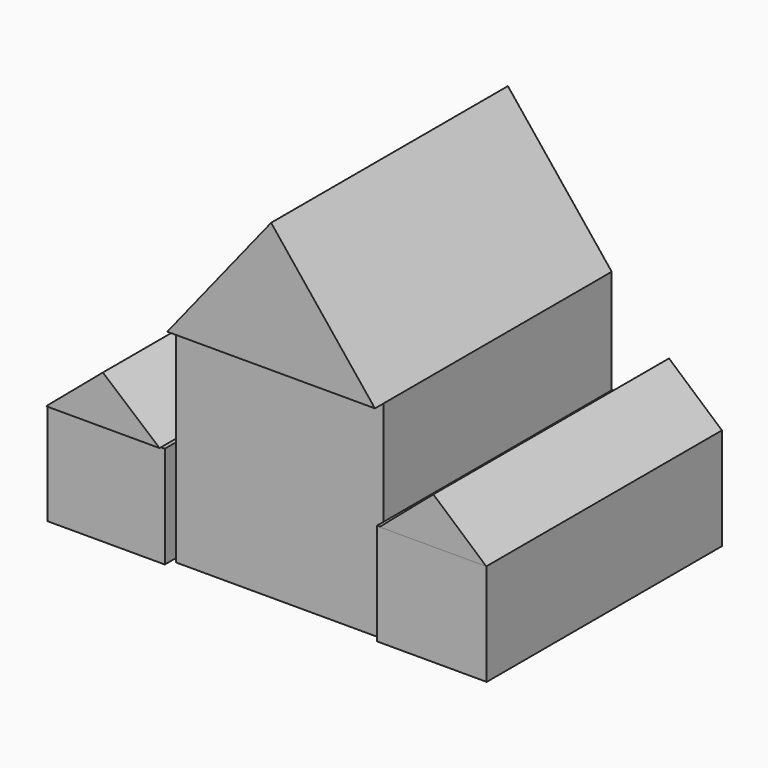
from build123d import *

# Parameters (mm, degrees)
F0_W      = 63.5
F0_H      = 63.5
F1_DEPTH  = 90.51564
F3_W      = 10.2954022586
F3_H      = 21.1791172624
F4_DEPTH  = 1.27
F6_W      = 6.7655518651
F6_H      = 6.3243201002
F7_DEPTH  = 5.08
F8_W      = 35.8868353069
F8_H      = 31.1803687364
F9_DEPTH  = 90.5202
F12_W     = 33.533602953
F12_H     = 31.1803687364
F13_DEPTH = 89.9029
F17_DEPTH = 90.07895
F19_DEPTH = 91.04824
F2_W      = 63.5
F2_H      = 63.5
F22_DEPTH = 3.36136


# Not quite as in the source:
# - the program builds the solid bodies; features that only make, move or delete a surface that nothing else refers to are left out


with BuildPart() as f1:
    # F0 (on Front) → F1 (new body)
    with BuildSketch(Plane.XZ):
        Polygon((-31.75, 31.75), (31.75, 31.75), (0, 71.4057372898), align=None)
        Rectangle(F0_W, F0_H)
    extrude(amount=F1_DEPTH)

    # F3 (on face) → F4 (cut)
    with BuildSketch(Plane.XZ.offset(90.51564)):
        with Locations((0, -20.0025010854)):
            Rectangle(F3_W, F3_H)
    extrude(amount=-F4_DEPTH, mode=Mode.SUBTRACT)

    # F6 (on face) → F7 (cut)
    with BuildSketch(Plane(origin=(-31.75, 0, 0), x_dir=(0, -1, 0), z_dir=(-1, 0, 0))):
        with Locations((15.6882982701, 15.3695684858)):
            Rectangle(F6_W, F6_H)
        with Locations((22.4538501352, 15.3695684858)):
            Rectangle(F6_W, F6_H)
        with Locations((22.4538501352, 9.0452483855)):
            Rectangle(F6_W, F6_H)
        with Locations((15.6882982701, 9.0452483855)):
            Rectangle(F6_W, F6_H)
    extrude(amount=-F7_DEPTH, mode=Mode.SUBTRACT)

    # F2 (on face) → F22 (cut)
    with BuildSketch(Plane.XZ.offset(90.51564)):
        Rectangle(F2_W, F2_H)
    extrude(amount=-F22_DEPTH, mode=Mode.SUBTRACT)


with BuildPart() as f9:
    # F8 (on Front) → F9 (new body)
    with BuildSketch(Plane.XZ):
        with Locations((-50.4474807531, -15.5901843682)):
            Rectangle(F8_W, F8_H)
    extrude(amount=F9_DEPTH)

    # F18 (on Front) → F19 (join)
    with BuildSketch(Plane.XZ):
        Polygon((-51.0357916355, 14.7077208385), (-68.3908984065, 0), (-33.6806811392, 0), align=None)
    extrude(amount=F19_DEPTH)


with BuildPart() as f13:
    # F12 (on Front) → F13 (new body)
    with BuildSketch(Plane.XZ):
        with Locations((48.6825555563, -15.5901843682)):
            Rectangle(F12_W, F12_H)
    extrude(amount=F13_DEPTH)

    # F16 (on Front) → F17 (join)
    with BuildSketch(Plane.XZ):
        Polygon((32.7982157469, 0), (65.4493570328, 0), (49.2708645761, 14.11941275), align=None)
    extrude(amount=F17_DEPTH)


solid = Compound([f1.part, f9.part, f13.part])
